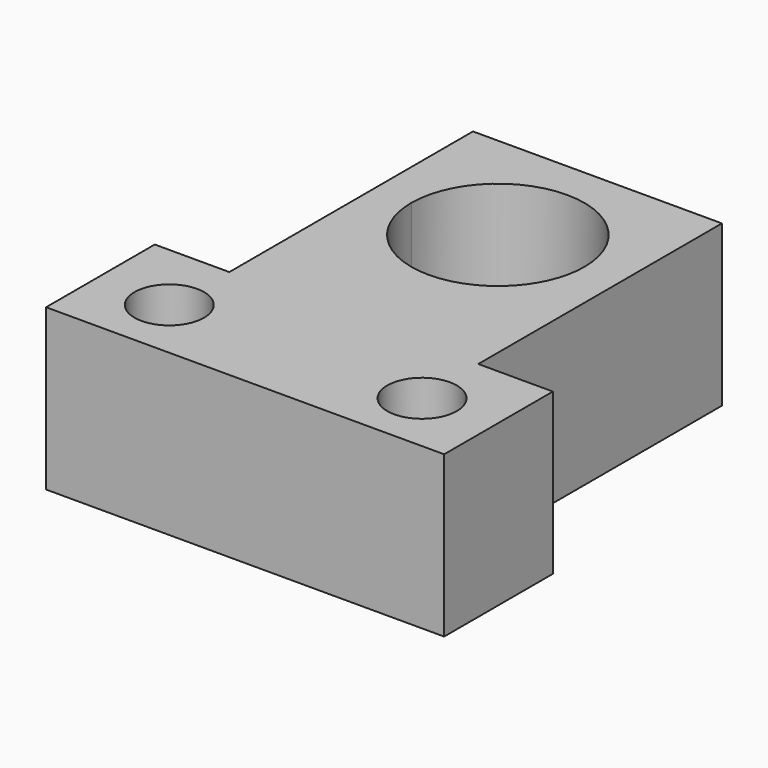
from build123d import *

# Parameters (mm, degrees)
F0_R     = 2.75
F0_W     = 1.85
F0_H     = 10.75
F0_W_2   = 10
F1_DEPTH = 12.7


# Not quite as in the source:
# - a length typed as a fraction of an inch, garbled in the dataset ("3 / 203.2 mm" for 3/8 in), is restored


with BuildPart() as f1:
    # F0 (on Top) → F1 (new body)
    with BuildSketch(Plane.XY):
        Polygon((-15.75, -14.25), (-15.75, -25), (-6.85, -25), (-6.85, -14.25), (-9.85, -14.25), align=None)
        with Locations((-10, -20)):
            Circle(F0_R, mode=Mode.SUBTRACT)
        with Locations((-5.925, -19.625)):
            Rectangle(F0_W, F0_H)
        with Locations((0, -19.625)):
            Rectangle(F0_W_2, F0_H)
        with BuildLine():
            Line((-9.85, -14.25), (-6.85, -14.25))
            Line((-6.85, -14.25), (-6.85, 0))
            ThreePointArc((-6.85, 0), (0, 6.85), (6.85, 0))
            Line((6.85, 0), (6.85, -14.25))
            Line((6.85, -14.25), (9.85, -14.25))
            Line((9.85, -14.25), (9.85, 9.85))
            Line((9.85, 9.85), (-9.85, 9.85))
            Line((-9.85, 9.85), (-9.85, -14.25))
        make_face()
        with Locations((5.925, -19.625)):
            Rectangle(F0_W, F0_H)
        Polygon((6.85, -14.25), (6.85, -25), (15.75, -25), (15.75, -14.25), (9.85, -14.25), align=None)
        with Locations((10, -20)):
            Circle(F0_R, mode=Mode.SUBTRACT)
        with BuildLine():
            Line((-6.85, 0), (-6.85, -14.25))
            Line((-6.85, -14.25), (-5, -14.25))
            Line((-5, -14.25), (-5, -4.6821469434))
            ThreePointArc((-5, -4.6821469434), (-6.3707338667, -2.5171908946), (-6.85, 0))
        make_face()
        with BuildLine():
            Line((5, -4.6821469434), (5, -14.25))
            Line((5, -14.25), (6.85, -14.25))
            Line((6.85, -14.25), (6.85, 0))
            ThreePointArc((6.85, 0), (6.3707338667, -2.5171908946), (5, -4.6821469434))
        make_face()
        with BuildLine():
            Line((-5, -4.6821469434), (-5, -14.25))
            Line((-5, -14.25), (5, -14.25))
            Line((5, -14.25), (5, -4.6821469434))
            ThreePointArc((5, -4.6821469434), (0, -6.85), (-5, -4.6821469434))
        make_face()
    extrude(amount=-F1_DEPTH)


solid = f1.part
